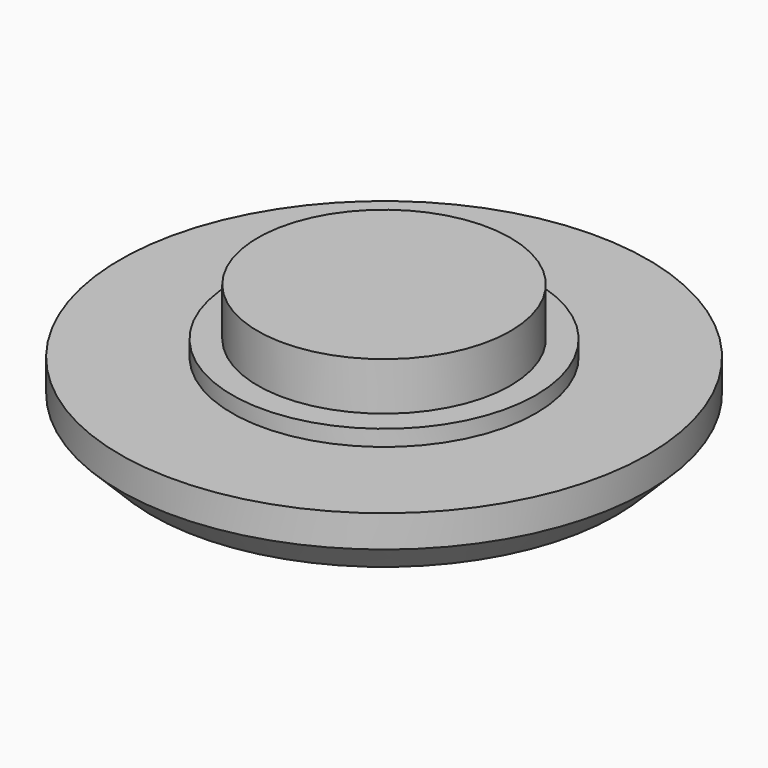
from build123d import *

# Parameters (mm, degrees)
F0_R     = 3.95
F1_DEPTH = 2
F0_R_2   = 8.25
F0_R_3   = 4.75
F2_DEPTH = 2
F3_DEPTH = 0.5
F4_SIZE  = 1


with BuildPart() as f1:
    # F0 (on Top) → F1 (new body)
    with BuildSketch(Plane.XY):
        Circle(F0_R)
    extrude(amount=F1_DEPTH)


with BuildPart() as f2:
    # F0 (on Top) → F2 (new body)
    with BuildSketch(Plane.XY):
        Circle(F0_R_2)
        Circle(F0_R_3, mode=Mode.SUBTRACT)
        Circle(F0_R_3)
        Circle(F0_R, mode=Mode.SUBTRACT)
        Circle(F0_R)
    extrude(amount=-F2_DEPTH)

    # F0 (on Top) → F3 (join)
    with BuildSketch(Plane.XY):
        Circle(F0_R_3)
        Circle(F0_R, mode=Mode.SUBTRACT)
        Circle(F0_R)
    extrude(amount=F3_DEPTH)

    # F4
    f4_edges = [f2.edges().sort_by_distance(p)[0] for p in [
        (-8.25, 0, -2),
    ]]
    chamfer(f4_edges, length=F4_SIZE)


solid = Compound([f1.part, f2.part])
